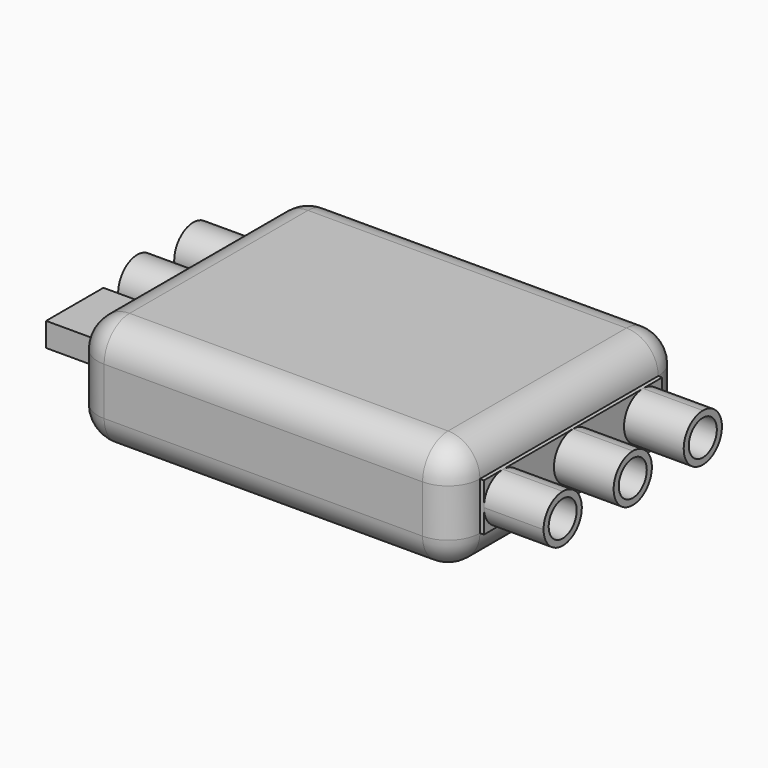
from build123d import *

# Parameters (mm, degrees)
F1_DEPTH  = 7
F2_R      = 2
F3_R      = 1.1
F4_DEPTH  = 4
F5_R      = 1.5
F5_R_2    = 1.1
F5_W      = 4.5
F5_H      = 1.5
F6_DEPTH  = 4
F7_W      = 14
F7_H      = 3
F8_DEPTH  = 0.25
F9_W      = 14
F9_H      = 3
F9_R      = 1.1
F10_DEPTH = 0.25


with BuildPart() as f1:
    # F0 (on Top) → F1 (new body)
    with BuildSketch(Plane.XY):
        with BuildLine():
            ThreePointArc((12, 7), (11.4142135624, 8.4142135624), (10, 9))
            Line((10, 9), (-10, 9))
            ThreePointArc((-10, 9), (-11.4142135624, 8.4142135624), (-12, 7))
            Line((-12, 7), (-12, -7))
            ThreePointArc((-12, -7), (-11.4142135624, -8.4142135624), (-10, -9))
            Line((-10, -9), (10, -9))
            ThreePointArc((10, -9), (11.4142135624, -8.4142135624), (12, -7))
            Line((12, -7), (12, 7))
        make_face()
    extrude(amount=F1_DEPTH)

    # F2
    f2_edges = [f1.edges().sort_by_distance(p)[0] for p in [
        (11.414214, 8.414214, 7),
        (0, 9, 7),
        (-11.414214, 8.414214, 7),
        (-12, 0, 7),
        (-11.414214, -8.414214, 7),
        (0, -9, 7),
        (11.414214, -8.414214, 7),
        (12, 0, 7),
        (11.414214, 8.414214, 0),
        (0, 9, 0),
        (-11.414214, 8.414214, 0),
        (-12, 0, 0),
        (-11.414214, -8.414214, 0),
        (0, -9, 0),
        (11.414214, -8.414214, 0),
        (12, 0, 0),
    ]]
    fillet(f2_edges, radius=F2_R)

    # F3 (on face) → F4 (join)
    with BuildSketch(Plane.YZ.offset(12)):
        with BuildLine():
            ThreePointArc((-4, 3.5), (-4.4393398246, 4.5606601681), (-5.4999999897, 5))
            ThreePointArc((-5.4999999897, 5), (-6.5606601681, 4.5606601754), (-7, 3.5))
            ThreePointArc((-7, 3.5), (-6.5606601718, 2.4393398282), (-5.5, 2))
            ThreePointArc((-5.5, 2), (-4.4393398282, 2.4393398282), (-4, 3.5))
        make_face()
        with Locations((-5.5, 3.5)):
            Circle(F3_R, mode=Mode.SUBTRACT)
        with BuildLine():
            ThreePointArc((0, 2), (1.0606601718, 2.4393398282), (1.5, 3.5))
            ThreePointArc((1.5, 3.5), (1.0606601718, 4.5606601718), (0, 5))
            ThreePointArc((0, 5), (-1.5, 3.5), (0, 2))
        make_face()
        with Locations((0, 3.5)):
            Circle(F3_R, mode=Mode.SUBTRACT)
        with BuildLine():
            ThreePointArc((7, 3.5), (6.5606601718, 4.5606601718), (5.5, 5))
            ThreePointArc((5.5, 5), (4, 3.499999998), (5.5000000039, 2))
            ThreePointArc((5.5000000039, 2), (6.5606601732, 2.4393398296), (7, 3.5))
        make_face()
        with Locations((5.5, 3.5)):
            Circle(F3_R, mode=Mode.SUBTRACT)
    extrude(amount=F4_DEPTH)

    # F5 (on face) → F6 (join)
    with BuildSketch(Plane(origin=(-12, 0, 0), x_dir=(0, -1, 0), z_dir=(-1, 0, 0))):
        with Locations((-5.5, 3.5)):
            Circle(F5_R)
        with Locations((-5.5, 3.5)):
            Circle(F5_R_2, mode=Mode.SUBTRACT)
        with Locations((-1.1, 3.5)):
            Circle(F5_R)
        with Locations((-1.1, 3.5)):
            Circle(F5_R_2, mode=Mode.SUBTRACT)
        with Locations((3.8085386623, 3.5)):
            Rectangle(F5_W, F5_H)
    extrude(amount=F6_DEPTH)

    # F7 (on face) → F8 (join)
    with BuildSketch(Plane.YZ.offset(12)):
        with Locations((0, 3.5)):
            Rectangle(F7_W, F7_H)
    extrude(amount=F8_DEPTH)

    # F9 (on face) → F10 (join)
    with BuildSketch(Plane(origin=(-12, 0, 0), x_dir=(0, -1, 0), z_dir=(-1, 0, 0))):
        with Locations((0, 3.5)):
            Rectangle(F9_W, F9_H)
        with Locations((-1.1, 3.5)):
            Circle(F9_R, mode=Mode.SUBTRACT)
        with Locations((-1.1, 3.5)):
            Circle(F9_R)
    extrude(amount=F10_DEPTH)


solid = f1.part
